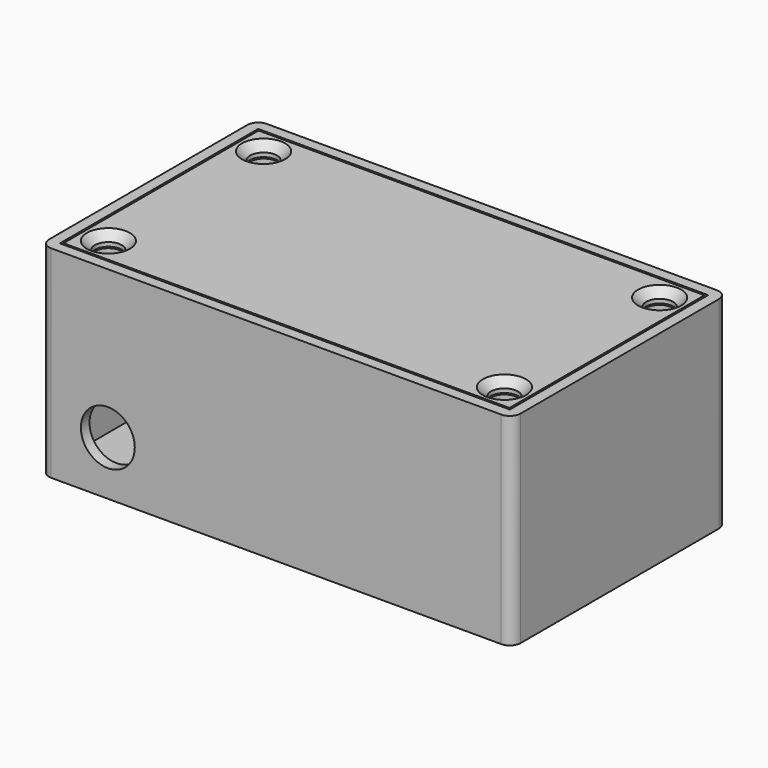
from build123d import *

# Parameters (mm, degrees)
F0_W        = 70
F0_H        = 40
F1_DEPTH    = 30
F2_T        = -1.6
F4_W        = 8
F4_H        = 8
F4_R        = 2
F5_DEPTH    = 10
F6_T1_DEPTH = 28.5734639037
F6_T3_DEPTH = 28.5734639037
F7_R        = 4
F8_DEPTH    = 25
F9_W        = 66.2
F9_H        = 36.2
F9_R        = 2
F10_DEPTH   = 1.8
F11_SIZE    = 1.2
F12_R       = 1.6


# Not quite as in the source:
# - a fillet or chamfer that OpenCascade refuses, or shapes differently, is made with other operations: its cross-section is extruded or revolved along the edge and cut away or added


with BuildPart() as f1:
    # F0 (on Top) → F1 (new body)
    with BuildSketch(Plane.XY):
        with Locations((-35, 20)):
            Rectangle(F0_W, F0_H)
    extrude(amount=F1_DEPTH)

    # F2
    f2_openings = [f1.faces().sort_by_distance(p)[0] for p in [
        (-35, 20, 30),
    ]]
    offset(amount=F2_T, openings=f2_openings)

    # F4 (on offset) → F5 (join)
    with BuildSketch(Plane.XY.offset(28)):
        with Locations((-64.4, 34.4)):
            Rectangle(F4_W, F4_H)
        with Locations((-64.4, 34.4)):
            Circle(F4_R, mode=Mode.SUBTRACT)
        with Locations((-5.6, 34.4)):
            Rectangle(F4_W, F4_H)
        with Locations((-5.6, 34.4)):
            Circle(F4_R, mode=Mode.SUBTRACT)
        with Locations((-64.4, 5.6)):
            Rectangle(F4_W, F4_H)
        with Locations((-64.4, 5.6)):
            Circle(F4_R, mode=Mode.SUBTRACT)
        with Locations((-5.6, 5.6)):
            Rectangle(F4_W, F4_H)
        with Locations((-5.6, 5.6)):
            Circle(F4_R, mode=Mode.SUBTRACT)
    extrude(amount=-F5_DEPTH)

    # F6: chamfer of 8 on 4 edges, made by hand

    # F6_s2 → F6_t1 (cut)
    with BuildSketch(Plane.XZ.offset(-38.4)):
        Polygon((-68.4, 18), (-60.4, 26), (-60.4, 18), align=None)
        Polygon((-9.6, 26), (-1.6, 18), (-9.6, 18), align=None)
    extrude(amount=F6_T1_DEPTH, mode=Mode.SUBTRACT)

    # F6_s4 → F6_t3 (cut)
    with BuildSketch(Plane.XZ.offset(-30.1734639037)):
        Polygon((-60.4, 26), (-68.4, 18), (-60.4, 18), align=None)
        Polygon((-1.6, 18), (-9.6, 26), (-9.6, 18), align=None)
    extrude(amount=F6_T3_DEPTH, mode=Mode.SUBTRACT)

    # F7 (on face) → F8 (cut)
    with BuildSketch(Plane.XZ):
        with Locations((-60, 8)):
            Circle(F7_R)
    extrude(amount=-F8_DEPTH, mode=Mode.SUBTRACT)

    # F12
    f12_edges = [f1.edges().sort_by_distance(p)[0] for p in [
        (-70, 0, 15),
        (-70, 40, 15),
        (0, 0, 15),
        (0, 40, 15),
    ]]
    fillet(f12_edges, radius=F12_R)


with BuildPart() as f10:
    # F9 (on face) → F10 (new body)
    with BuildSketch(Plane.XY.offset(30)):
        with Locations((-35, 20)):
            Rectangle(F9_W, F9_H)
        with Locations((-64.4, 5.6)):
            Circle(F9_R, mode=Mode.SUBTRACT)
        with Locations((-5.6, 5.6)):
            Circle(F9_R, mode=Mode.SUBTRACT)
        with Locations((-64.4, 34.4)):
            Circle(F9_R, mode=Mode.SUBTRACT)
        with Locations((-5.6, 34.4)):
            Circle(F9_R, mode=Mode.SUBTRACT)
    extrude(amount=-F10_DEPTH)

    # F11
    f11_edges = [f10.edges().sort_by_distance(p)[0] for p in [
        (-7.6, 5.6, 30),
        (-66.4, 5.6, 30),
        (-66.4, 34.4, 30),
        (-7.6, 34.4, 30),
    ]]
    chamfer(f11_edges, length=F11_SIZE)


solid = Compound([f1.part, f10.part])
